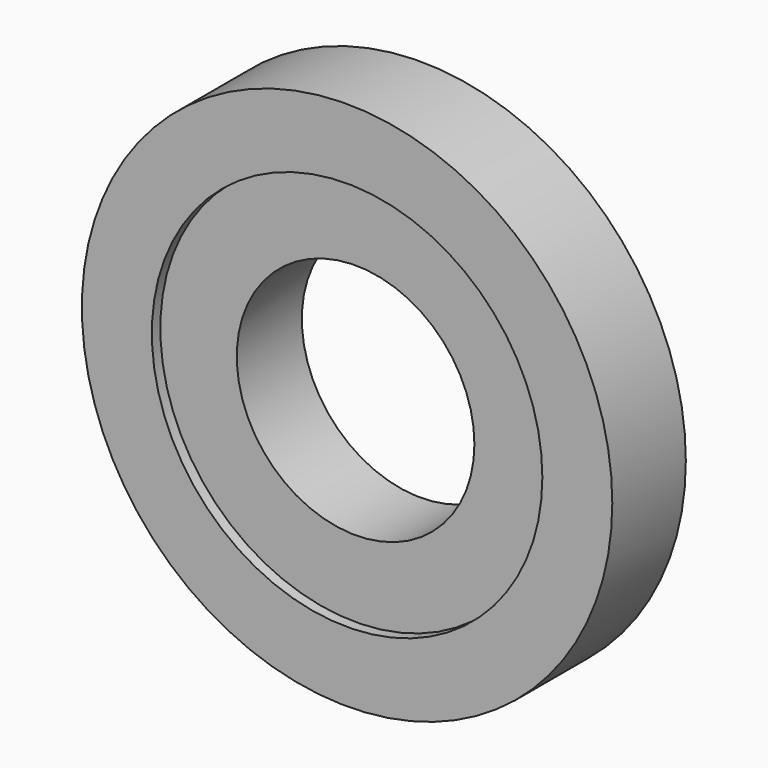
from build123d import *

# Parameters (mm, degrees)
F0_R     = 19.05
F1_DEPTH = 3.302
F2_R     = 8.5345501525
F3_DEPTH = 6.605
F4_R     = 14.0253085835
F4_R_2   = 8.5345501525
F5_DEPTH = 0.762


# Not quite as in the source:
# - a feature names something its author has since deleted; it is built from what else it names


with BuildPart() as f1:
    # F0 (on Front) → F1 (new body, symmetric)
    with BuildSketch(Plane.XZ):
        Circle(F0_R)
    extrude(amount=F1_DEPTH, both=True)

    # F2 (on face) → F3 (cut, through all)
    with BuildSketch(Plane.XZ.offset(3.302)):
        Circle(F2_R)
    extrude(amount=-F3_DEPTH, mode=Mode.SUBTRACT)

    # F4 (on face) → F5 (cut)
    with BuildSketch(Plane.XZ.offset(3.302)):
        Circle(F4_R)
        Circle(F4_R_2, mode=Mode.SUBTRACT)
    extrude(amount=-F5_DEPTH, mode=Mode.SUBTRACT)


solid = f1.part
